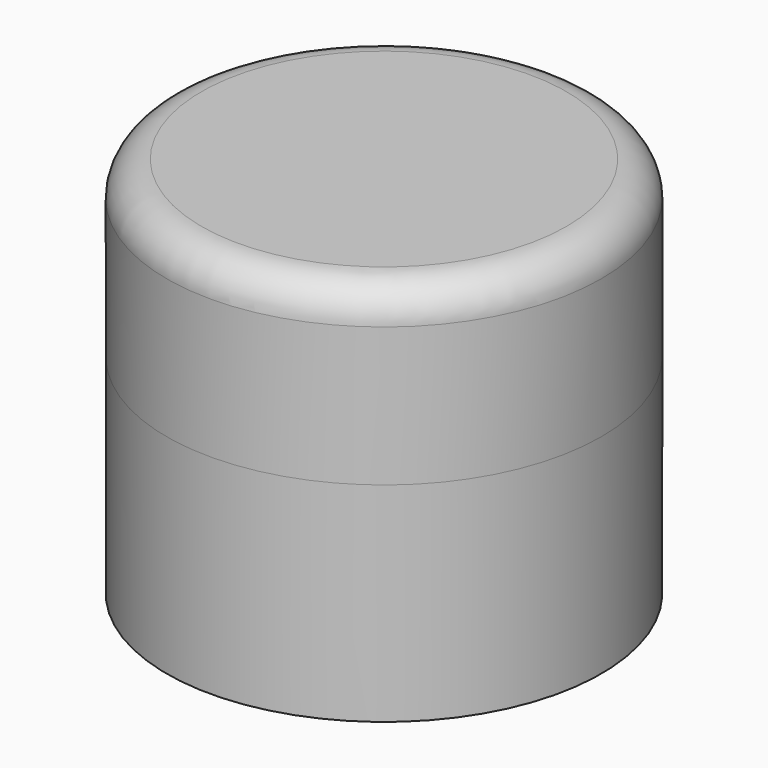
from build123d import *

# Parameters (mm, degrees)
F0_R     = 3.048
F1_DEPTH = 7.62
F2_W     = 6.604
F2_H     = 1.016
F3_DEPTH = 2.54
F4_R     = 7.9375
F5_DEPTH = 6.35


# Not quite as in the source:
# - a fillet or chamfer that OpenCascade refuses, or shapes differently, is made with other operations: its cross-section is extruded or revolved along the edge and cut away or added


with BuildPart() as f1:
    # F0 (on Top) → F1 (new body)
    with BuildSketch(Plane.XY):
        with BuildLine():
            Line((0, 10.275801), (-1.778, 7.735801))
            ThreePointArc((-1.778, 7.735801), (0, -7.9375), (1.778, 7.735801))
            Line((1.778, 7.735801), (0, 10.275801))
        make_face()
        Circle(F0_R, mode=Mode.SUBTRACT)
    extrude(amount=F1_DEPTH)

    # F2 (on face) → F3 (join)
    with BuildSketch(Plane.XY.offset(7.62)):
        Rectangle(F2_W, F2_H)
    extrude(amount=-F3_DEPTH)

    # F4 (on face) → F5 (join)
    with BuildSketch(Plane.XY.offset(7.62)):
        Circle(F4_R)
    extrude(amount=F5_DEPTH)

    # F6 (on Right) → F7 (revolve, cut)
    with BuildSketch(Plane.YZ):
        Polygon((10.275801, 8.165955), (7.9375, 8.165955), (7.9375, 4.064), (10.275801, 2.286), align=None)
    revolve(axis=Axis((0, 0, 8.534907), (0, 0, 1)), mode=Mode.SUBTRACT)

    # F8: fillet of radius 1.27 on 1 edges, made by hand

    # F8_s1 → F8_t2 (revolve, cut)
    with BuildSketch(Plane.XZ):
        with BuildLine():
            ThreePointArc((7.9375, 12.7), (7.565526, 13.598026), (6.6675, 13.97))
            Line((6.6675, 13.97), (7.9375, 13.97))
            Line((7.9375, 13.97), (7.9375, 12.7))
        make_face()
    revolve(axis=Axis((0, 0, 13.97), (0, 0, 1)), mode=Mode.SUBTRACT)


solid = f1.part
